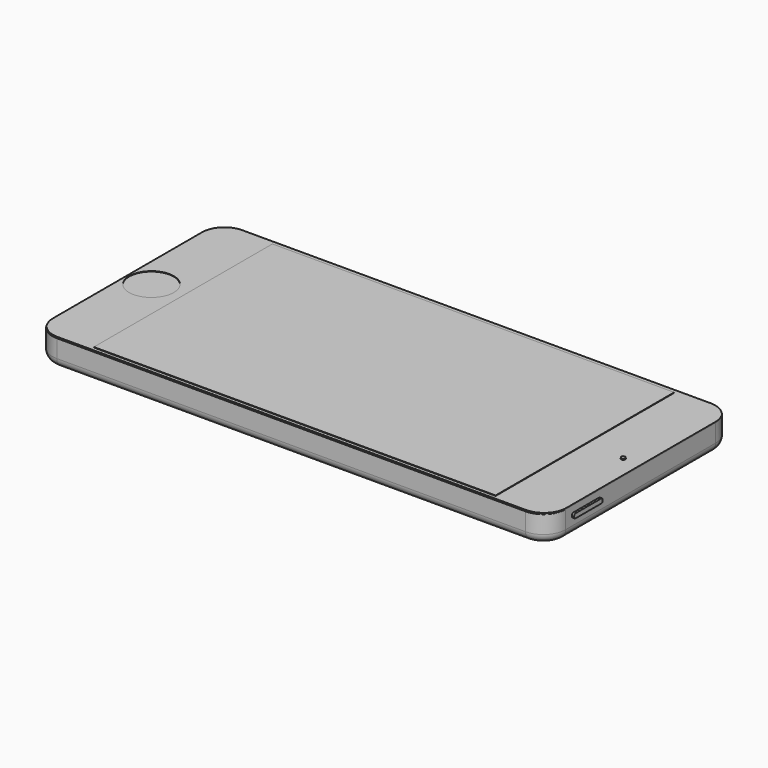
from build123d import *

# Parameters (mm, degrees)
F0_W         = 115
F0_H         = 52
F1_DEPTH     = 6
F2_R         = 5
F3_R         = 5
F4_R         = 5
F5_R         = 5
F6_R         = 2
F7_W         = 7
F7_H         = 1
F8_DEPTH     = 0.5
F9_R         = 0.4
F10_W        = 8
F10_H        = 1
F11_DEPTH    = 0.5
F12_R        = 0.4
F13_R        = 1.3753427914
F14_DEPTH    = 5
F15_W        = 7.2263174225
F15_H        = 1.4154640958
F16_DEPTH    = 5
F17_T1_DEPTH = 7.25
F18_R        = 0.4599630822
F18_R_2      = 0.4249345938
F18_R_3      = 0.4227374369
F18_R_4      = 0.410570945
F18_R_5      = 0.3795025996
F19_DEPTH    = 1
F20_W        = 8
F20_H        = 1
F21_DEPTH    = 0.5
F22_R        = 0.4
F23_R        = 3
F23_R_2      = 1.4921578392
F24_DEPTH    = 0.5
F25_W        = 1
F25_H        = 1.5
F26_DEPTH    = 0.5
F27_R        = 0.49999
F28_R        = 1.75
F29_DEPTH    = 1
F30_R        = 0.99999
F31_W        = 7
F31_H        = 21
F32_DEPTH    = 0.1
F33_R        = 3
F34_W        = 115
F34_H        = 51.7527479678
F35_DEPTH    = 0.2
F36_R        = 5
F38_R        = 0.5
F39_DEPTH    = 0.2
F40_W        = 90
F40_H        = 50
F41_DEPTH    = 0.1
F42_R        = 5
F43_DEPTH    = 0.1


# Not quite as in the source:
# - a fillet or chamfer that OpenCascade refuses, or shapes differently, is made with other operations: its cross-section is extruded or revolved along the edge and cut away or added
# - a fillet or chamfer is up to 0.001 mm smaller than in the source, because OpenCascade refuses the exact size


with BuildPart() as f1:
    # F0 (on Top) → F1 (new body)
    with BuildSketch(Plane.XY):
        Rectangle(F0_W, F0_H)
    extrude(amount=F1_DEPTH)

    # F2
    f2_edges = [f1.edges().sort_by_distance(p)[0] for p in [
        (57.5, 26, 3),
    ]]
    fillet(f2_edges, radius=F2_R)

    # F3
    f3_edges = [f1.edges().sort_by_distance(p)[0] for p in [
        (57.5, -26, 3),
    ]]
    fillet(f3_edges, radius=F3_R)

    # F4
    f4_edges = [f1.edges().sort_by_distance(p)[0] for p in [
        (-57.5, -26, 3),
    ]]
    fillet(f4_edges, radius=F4_R)

    # F5
    f5_edges = [f1.edges().sort_by_distance(p)[0] for p in [
        (-57.5, 26, 3),
    ]]
    fillet(f5_edges, radius=F5_R)

    # F6
    f6_edges = [f1.edges().sort_by_distance(p)[0] for p in [
        (0, -26, 0),
    ]]
    fillet(f6_edges, radius=F6_R)

    # F7 (on face) → F8 (join)
    with BuildSketch(Plane(origin=(0, 26, 0), x_dir=(-1, 0, 0), z_dir=(0, 1, 0))):
        with Locations((-39.7966161668, 4.1244386885)):
            Rectangle(F7_W, F7_H)
    extrude(amount=F8_DEPTH)

    # F9
    f9_edges = [f1.edges().sort_by_distance(p)[0] for p in [
        (43.296616, 26.25, 4.624439),
        (43.296616, 26.25, 3.624439),
        (36.296616, 26.25, 3.624439),
        (36.296616, 26.25, 4.624439),
    ]]
    fillet(f9_edges, radius=F9_R)

    # F10 (on face) → F11 (join)
    with BuildSketch(Plane(origin=(0, 26, 0), x_dir=(-1, 0, 0), z_dir=(0, 1, 0))):
        with Locations((-30.6172464043, 4.2625843126)):
            Rectangle(F10_W, F10_H)
    extrude(amount=F11_DEPTH)

    # F12
    f12_edges = [f1.edges().sort_by_distance(p)[0] for p in [
        (34.617246, 26.25, 4.762584),
        (34.617246, 26.25, 3.762584),
        (26.617246, 26.25, 3.762584),
        (26.617246, 26.25, 4.762584),
    ]]
    fillet(f12_edges, radius=F12_R)

    # F13 (on face) → F14 (cut)
    with BuildSketch(Plane(origin=(-57.5, 0, 0), x_dir=(0, -1, 0), z_dir=(-1, 0, 0))):
        with Locations((-18.6263173819, 3.5008231644)):
            Circle(F13_R)
    extrude(amount=-F14_DEPTH, mode=Mode.SUBTRACT)

    # F15 (on face) → F16 (cut)
    with BuildSketch(Plane(origin=(-57.5, 0, 0), x_dir=(0, -1, 0), z_dir=(-1, 0, 0))):
        with Locations((-0.1417595195, 3.6792070605)):
            Rectangle(F15_W, F15_H)
    extrude(amount=-F16_DEPTH, mode=Mode.SUBTRACT)

    # F17: fillet of radius 0.9 on 4 edges, made by hand

    # F17_s2 → F17_t1 (join)
    with BuildSketch(Plane.YZ.offset(-57.5)):
        with BuildLine():
            ThreePointArc((3.7549182307, 3.4869391084), (3.4913143338, 4.1233352114), (2.8549182307, 4.3869391084))
            Line((2.8549182307, 4.3869391084), (3.7549182307, 4.3869391084))
            Line((3.7549182307, 4.3869391084), (3.7549182307, 3.4869391084))
        make_face()
        with BuildLine():
            ThreePointArc((2.8549182307, 2.9714750126), (3.4913143338, 3.2350789095), (3.7549182307, 3.8714750126))
            Line((3.7549182307, 3.8714750126), (3.7549182307, 2.9714750126))
            Line((3.7549182307, 2.9714750126), (2.8549182307, 2.9714750126))
        make_face()
        with BuildLine():
            ThreePointArc((-3.4713991918, 3.4869391084), (-3.2077952948, 4.1233352114), (-2.5713991918, 4.3869391084))
            Line((-2.5713991918, 4.3869391084), (-3.4713991918, 4.3869391084))
            Line((-3.4713991918, 4.3869391084), (-3.4713991918, 3.4869391084))
        make_face()
        with BuildLine():
            ThreePointArc((-3.4713991918, 3.8714750126), (-3.2077952948, 3.2350789095), (-2.5713991918, 2.9714750126))
            Line((-2.5713991918, 2.9714750126), (-3.4713991918, 2.9714750126))
            Line((-3.4713991918, 2.9714750126), (-3.4713991918, 3.8714750126))
        make_face()
    extrude(amount=F17_T1_DEPTH)

    # F18 (on face) → F19 (cut)
    with BuildSketch(Plane(origin=(-57.5, 0, 0), x_dir=(0, -1, 0), z_dir=(-1, 0, 0))):
        with Locations((10.0176958367, 3.8720327429)):
            Circle(F18_R)
        with Locations((11.2625658512, 3.8720327429)):
            Circle(F18_R_2)
        with Locations((12.5212017447, 3.8720327429)):
            Circle(F18_R_3)
        with Locations((13.5920578614, 3.8720327429)):
            Circle(F18_R_4)
        with Locations((14.7436074913, 3.8720327429)):
            Circle(F18_R_5)
    extrude(amount=-F19_DEPTH, mode=Mode.SUBTRACT)

    # F20 (on face) → F21 (join)
    with BuildSketch(Plane.YZ.offset(57.5)):
        with Locations((-15.2602228336, 4.0141151957)):
            Rectangle(F20_W, F20_H)
    extrude(amount=F21_DEPTH)

    # F22
    f22_edges = [f1.edges().sort_by_distance(p)[0] for p in [
        (57.75, -19.260223, 4.514115),
        (57.75, -19.260223, 3.514115),
        (57.75, -11.260223, 4.514115),
        (57.75, -11.260223, 3.514115),
    ]]
    fillet(f22_edges, radius=F22_R)

    # F25 (on face) → F26 (cut)
    with BuildSketch(Plane(origin=(0, 0, 0), x_dir=(1, 0, 0), z_dir=(0, 0, -1))):
        with Locations((51.1113621431, 14.2942524761)):
            Rectangle(F25_W, F25_H)
    extrude(amount=-F26_DEPTH, mode=Mode.SUBTRACT)

    # F27 (radius 0.5 in the source; OpenCascade refuses exactly that, so slightly less here)
    f27_edges = [f1.edges().sort_by_distance(p)[0] for p in [
        (50.611362, -13.544252, 0.25),
        (50.611362, -15.044252, 0.25),
        (51.611362, -15.044252, 0.25),
        (51.611362, -13.544252, 0.25),
    ]]
    fillet(f27_edges, radius=F27_R)

    # F28 (on face) → F29 (cut)
    with BuildSketch(Plane(origin=(0, 0, 0), x_dir=(1, 0, 0), z_dir=(0, 0, -1))):
        with Locations((51.2039475143, 9.4451671466)):
            Circle(F28_R)
    extrude(amount=-F29_DEPTH, mode=Mode.SUBTRACT)

    # F30 (radius 1 in the source; OpenCascade refuses exactly that, so slightly less here)
    f30_edges = [f1.edges().sort_by_distance(p)[0] for p in [
        (49.453948, -9.445167, 1),
    ]]
    fillet(f30_edges, radius=F30_R)


with BuildPart() as f24:
    # F23 (on face) → F24 (new body)
    with BuildSketch(Plane(origin=(0, 0, 0), x_dir=(1, 0, 0), z_dir=(0, 0, -1))):
        with Locations((51.158413291, 20.04163526)):
            Circle(F23_R)
        with Locations((51.158413291, 20.04163526)):
            Circle(F23_R_2, mode=Mode.SUBTRACT)
    extrude(amount=F24_DEPTH)


with BuildPart() as f32:
    # F31 (on face) → F32 (new body)
    with BuildSketch(Plane(origin=(0, 0, 0), x_dir=(1, 0, 0), z_dir=(0, 0, -1))):
        with Locations((48.0644905215, -10.4159945622)):
            Rectangle(F31_W, F31_H)
    extrude(amount=F32_DEPTH)

    # F33
    f33_edges = [f32.edges().sort_by_distance(p)[0] for p in [
        (51.564491, 20.915995, -0.05),
        (44.564491, 20.915995, -0.05),
        (51.564491, -0.084005, -0.05),
        (44.564491, -0.084005, -0.05),
    ]]
    fillet(f33_edges, radius=F33_R)


with BuildPart() as f35:
    # F34 (on face) → F35 (new body)
    with BuildSketch(Plane.XY.offset(6)):
        with Locations((0, 0.0527398661)):
            Rectangle(F34_W, F34_H)
    extrude(amount=F35_DEPTH)

    # F36
    f36_edges = [f35.edges().sort_by_distance(p)[0] for p in [
        (-57.5, 25.929114, 6.1),
        (57.5, 25.929114, 6.1),
        (57.5, -25.823634, 6.1),
        (-57.5, -25.823634, 6.1),
    ]]
    fillet(f36_edges, radius=F36_R)

    # F42 (on face) → F43 (cut)
    with BuildSketch(Plane.XY.offset(6.2)):
        with Locations((-52.0923775704, 0)):
            Circle(F42_R)
    extrude(amount=-F43_DEPTH, mode=Mode.SUBTRACT)


with BuildPart() as f39:
    # F38 (on face) → F39 (new body)
    with BuildSketch(Plane.XY.offset(6.2)):
        with Locations((53.5810078753, 0)):
            Circle(F38_R)
    extrude(amount=F39_DEPTH)


with BuildPart() as f41:
    # F40 (on face) → F41 (new body)
    with BuildSketch(Plane.XY.offset(6.2)):
        Rectangle(F40_W, F40_H)
    extrude(amount=F41_DEPTH)


solid = Compound([f1.part, f24.part, f32.part, f35.part, f39.part, f41.part])
